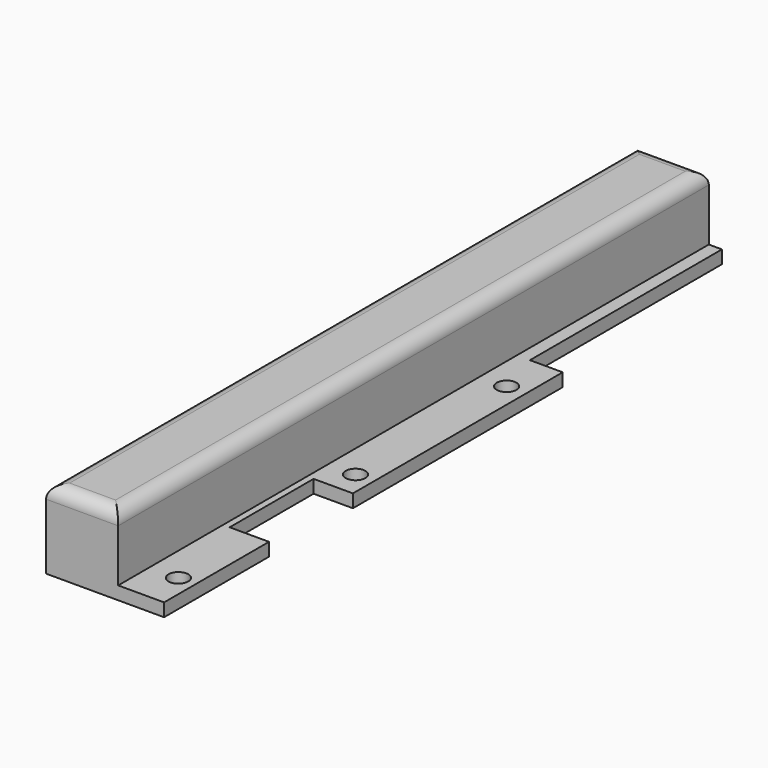
from build123d import *

# Parameters (mm, degrees)
F0_W     = 11
F0_H     = 112.6
F1_DEPTH = 2
F3_W     = 11
F3_H     = 112.6
F4_DEPTH = 10
F5_R     = 2
F6_R     = 1.5
F7_DEPTH = 25


with BuildPart() as f1:
    # F0 (on Top) → F1 (new body)
    with BuildSketch(Plane.XY):
        Polygon((-31.7652441872, 6.6397131595), (-31.7652441872, 43.2397131595), (-33.7652441872, 43.2397131595), (-33.7652441872, -69.3602868405), (-26.7652441872, -69.3602868405), (-26.7652441872, -49.3602868405), (-32.7652441872, -49.3602868405), (-32.7652441872, -33.3602868405), (-26.7652441872, -33.3602868405), (-26.7652441872, 6.6397131595), align=None)
        with Locations((-39.2652441872, -13.0602868405)):
            Rectangle(F0_W, F0_H)
    extrude(amount=F1_DEPTH)

    # F3 (on offset) → F4 (join)
    with BuildSketch(Plane.XY.offset(2)):
        with Locations((-39.2652441872, -13.0602868405)):
            Rectangle(F3_W, F3_H)
    extrude(amount=F4_DEPTH)

    # F5
    f5_edges = [f1.edges().sort_by_distance(p)[0] for p in [
        (-39.265244, 43.239713, 12),
        (-44.765244, -13.060287, 12),
        (-33.765244, -13.060287, 12),
        (-39.265244, -69.360287, 12),
    ]]
    fillet(f5_edges, radius=F5_R)

    # F6 (on face) → F7 (cut)
    with BuildSketch(Plane.XY.offset(2)):
        with Locations((-29.7272081302, -0.3602868405)):
            Circle(F6_R)
        with Locations((-29.5696301797, -29.3602868405)):
            Circle(F6_R)
        with Locations((-29.3848836171, -63.3602868405)):
            Circle(F6_R)
    extrude(amount=-F7_DEPTH, mode=Mode.SUBTRACT)


solid = f1.part
